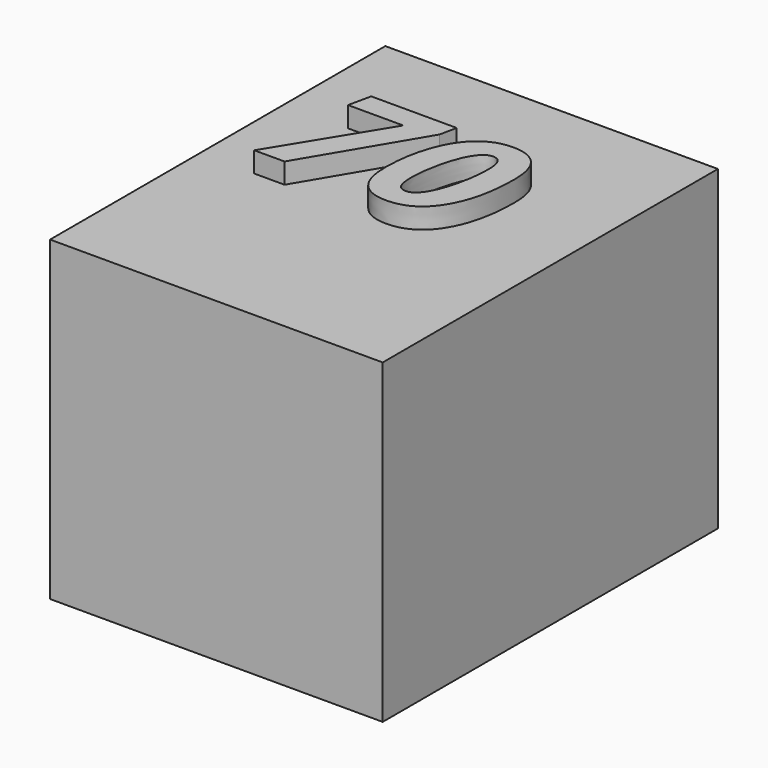
from build123d import *

# Parameters (mm, degrees)
F0_W          = 70.1691545546
F0_H          = 66.7628822848
F1_DEPTH      = 59.944
F2_W          = 70.1691545546
F2_H          = 66.7628822848
F3_DEPTH      = 25.4
F4_T          = -2.54
F5_W          = 70.1691545546
F5_H          = 66.7628822848
F6_DEPTH      = 3.048
F8_W          = 22.5326502696
F8_H          = 7.8291408718
F9_DEPTH      = 15.24
F10_TEXT_SIZE = 37.9130871604
F11_DEPTH     = 4.318


# Not quite as in the source:
# - Text() gives the source's letters only with a copy of the font that has no kerning and outlines rounded to 1/6400 em; it was checked with that copy


with BuildPart() as f1:
    # F0 (on Front) → F1 (new body)
    with BuildSketch(Plane.XZ):
        with Locations((3.3540148288, 18.6386168934)):
            Rectangle(F0_W, F0_H)
    extrude(amount=F1_DEPTH)

    # F2 (on face) → F3 (join)
    with BuildSketch(Plane(origin=(0, 0, 0), x_dir=(-1, 0, 0), z_dir=(0, 1, 0))):
        with Locations((-3.3540148288, 18.6386168934)):
            Rectangle(F2_W, F2_H)
    extrude(amount=F3_DEPTH)

    # F4
    f4_openings = [f1.faces().sort_by_distance(p)[0] for p in [
        (3.354015, 25.4, 18.638617),
    ]]
    offset(amount=F4_T, openings=f4_openings)

    # F5 (on face) → F6 (join)
    with BuildSketch(Plane(origin=(0, 25.4, 0), x_dir=(-1, 0, 0), z_dir=(0, 1, 0))):
        with Locations((-3.3540148288, 18.6386168934)):
            Rectangle(F5_W, F5_H)
    extrude(amount=F6_DEPTH)

    # F8 (on face) → F9 (cut)
    with BuildSketch(Plane(origin=(0, 28.448, 0), x_dir=(-1, 0, 0), z_dir=(0, 1, 0))):
        with Locations((-2.1005007438, 23.3919452876)):
            Rectangle(F8_W, F8_H)
    extrude(amount=-F9_DEPTH, mode=Mode.SUBTRACT)

    # F10 (on face) → F11 (join)
    with BuildSketch(Plane.XY.offset(52.0200580359)):
        with Locations((-21.6407878324, -20.5481210724)):
            Text('70', F10_TEXT_SIZE, font='Open Sans', font_style=FontStyle.BOLDITALIC, text_align=(TextAlign.LEFT, TextAlign.BOTTOM))
    extrude(amount=F11_DEPTH)


solid = f1.part
